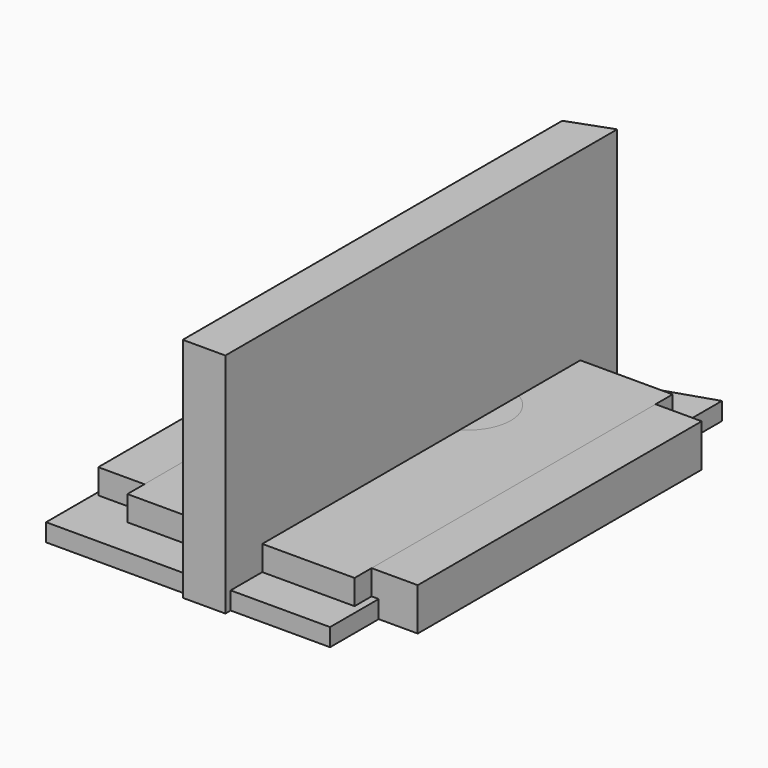
from build123d import *

# Parameters (mm, degrees)
F1_DEPTH  = 7.9375
F3_W      = 101.6
F3_H      = 88.9
F4_DEPTH  = 19.05
F6_DEPTH  = 101.6
F7_W      = 142.875
F7_H      = 158.75
F8_DEPTH  = 19.05
F10_DEPTH = 25.4
F11_R     = 5.08
F13_W     = 101.6
F13_H     = 177.8
F13_R     = 19.05
F14_DEPTH = 19.05
F15_R     = 4.92125
F16_DEPTH = 50.8


with BuildPart() as f1:
    # F0 (on Top) → F1 (new body)
    with BuildSketch(Plane.XY):
        Polygon((-73.0081277841, 71.2086516966), (-73.0081277841, -106.5913483034), (53.9918722159, -106.5913483034), (53.9918722159, 112.4836516966), align=None)
    extrude(amount=F1_DEPTH)


with BuildPart() as f2_1:
    # F2: copy of F1
    add(f1.part)


with BuildPart() as f4:
    # F3 (on Top) → F4 (new body)
    with BuildSketch(Plane.XY):
        Rectangle(F3_W, F3_H)
    extrude(amount=F4_DEPTH)


with BuildPart() as f6:
    # F5 (on Top) → F6 (new body)
    with BuildSketch(Plane.XY):
        Polygon((-9.525, 102.6038670372), (-9.525, -109.5375), (9.525, -109.5375), (9.525, 109.5375), align=None)
    extrude(amount=F6_DEPTH)


with BuildPart() as f8:
    # F7 (on Top) → F8 (new body)
    with BuildSketch(Plane.XY):
        Rectangle(F7_W, F7_H)
    extrude(amount=F8_DEPTH)


with BuildPart() as f10:
    # F9 (on Top) → F10 (new body)
    with BuildSketch(Plane.XY):
        Polygon((-39.9591773748, 42.2504134476), (-42.1587638557, -36.0182486475), (-18.8797935843, -39.1343310475), (-19.0630927682, 3.574329894), (9.8981438205, 17.5050515682), (20.5294843763, -29.9693830311), (55.5395893753, -21.9042263925), (59.022270143, 14.3889700994), (40.6923741102, 31.0691762716), (49.8573184013, 57.6475262642), align=None)
    extrude(amount=F10_DEPTH)

    # F11
    f11_edges = [f10.edges().sort_by_distance(p)[0] for p in [
        (-18.971443, -17.780001, 25.4),
        (-4.582474, 10.539691, 25.4),
        (15.213814, -6.232166, 25.4),
        (-41.058971, 3.116082, 25.4),
        (-30.519279, -37.57629, 25.4),
        (38.034537, -25.936805, 25.4),
        (57.28093, -3.757628, 25.4),
        (49.857322, 22.729073, 25.4),
        (45.274846, 44.358351, 25.4),
        (4.949071, 49.94897, 25.4),
    ]]
    fillet(f11_edges, radius=F11_R)


with BuildPart() as f14:
    # F13 (on Top) → F14 (new body)
    with BuildSketch(Plane.XY):
        Rectangle(F13_W, F13_H)
        with Locations((0, 38.1)):
            Circle(F13_R, mode=Mode.SUBTRACT)
    extrude(amount=F14_DEPTH)

    # F15 (on face) → F16 (join)
    with BuildSketch(Plane.XY.offset(19.05)):
        with Locations((-32.6851345599, -41.3269400597)):
            Circle(F15_R)
    extrude(amount=F16_DEPTH)


solid = Compound([f1.part, f2_1.part, f4.part, f6.part, f8.part, f14.part])
